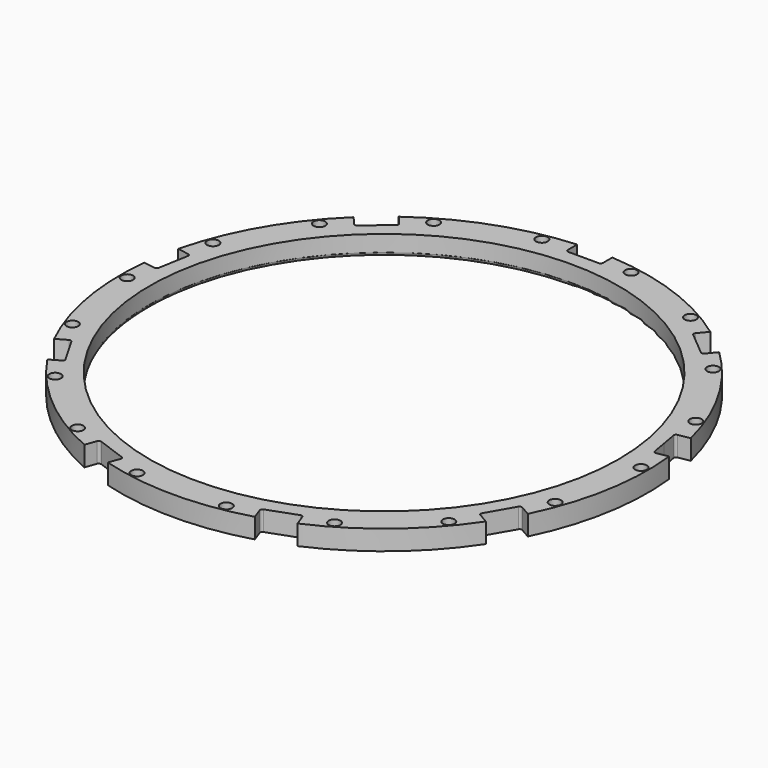
from build123d import *

# Parameters (mm, degrees)
F0_R           = 225
F0_R_2         = 200
F1_DEPTH       = 17
F3_D           = 5.5
F3_CBORE_D     = 10
F3_CBORE_DEPTH = 5.4
F4_R           = 3
F6_DEPTH       = 17.001


# Not quite as in the source:
# - a feature names something its author has since deleted; it is built from what else it names


with BuildPart() as f1:
    # F0 (on Top) → F1 (new body)
    with BuildSketch(Plane.XY):
        Circle(F0_R)
        Circle(F0_R_2, mode=Mode.SUBTRACT)
    extrude(amount=F1_DEPTH)

    # F3 (through all)
    with Locations(Plane.XY.offset(17)):
        with Locations((219, 0), (205.7926839521, 74.9024113883), (167.7637330431, 140.7704865214), (109.5, 189.6595634288), (38.0289509091, 215.6728979097), (-38.0289509091, 215.6728979097), (-109.5, 189.6595634288), (-167.7637330431, 140.7704865214), (-205.7926839521, 74.9024113883), (-219, 0), (-205.7926839521, -74.9024113883), (-167.7637330431, -140.7704865214), (-109.5, -189.6595634288), (-38.0289509091, -215.6728979097), (38.0289509091, -215.6728979097), (109.5, -189.6595634288), (167.7637330431, -140.7704865214), (205.7926839521, -74.9024113883)):
            CounterBoreHole(F3_D / 2, F3_CBORE_D / 2, F3_CBORE_DEPTH)

    # F4
    f4_edges = [f1.edges().sort_by_distance(p)[0] for p in [
        (-200, 0, 0),
    ]]
    fillet(f4_edges, radius=F4_R)

    # F5 (on face) → F6 (cut, through all)
    with BuildSketch(Plane.XY.offset(17)):
        with BuildLine():
            ThreePointArc((223.6935148816, 24.2118029049), (221.5817444277, 39.0708399751), (218.4840695516, 53.7560354952))
            Line((218.4840695516, 53.7560354952), (208.6359920215, 52.0195537186))
            ThreePointArc((208.6359920215, 52.0195537186), (207.3449842883, 51.1970910852), (207.0136728708, 49.7026418572))
            Line((207.0136728708, 49.7026418572), (209.2710991805, 36.900141068))
            Line((209.2710991805, 36.900141068), (211.5285254901, 24.0976402789))
            ThreePointArc((211.5285254901, 24.0976402789), (212.3509881235, 22.8066325456), (213.8454373515, 22.4753211282))
            Line((213.8454373515, 22.4753211282), (223.6935148816, 24.2118029049))
        make_face()
        with BuildLine():
            Line((149.3682510245, 154.6742923751), (155.7961271214, 162.3347368063))
            ThreePointArc((155.7961271214, 162.3347368063), (144.6272121795, 172.3599997018), (132.8147938278, 181.6183650969))
            Line((132.8147938278, 181.6183650969), (126.386917731, 173.9579206657))
            ThreePointArc((126.386917731, 173.9579206657), (125.926617221, 172.4980339608), (126.6334313978, 171.1402565601))
            Line((126.6334313978, 171.1402565601), (136.5920091584, 162.7840176342))
            Line((136.5920091584, 162.7840176342), (146.5505869189, 154.4277787082))
            ThreePointArc((146.5505869189, 154.4277787082), (148.0104736238, 153.9674781983), (149.3682510245, 154.6742923751))
        make_face()
        with BuildLine():
            Line((15, 214.4994432064), (15, 224.4994432064))
            ThreePointArc((15, 224.4994432064), (0, 225), (-15, 224.4994432064))
            Line((-15, 224.4994432064), (-15, 214.4994432064))
            ThreePointArc((-15, 214.4994432064), (-14.4142135624, 213.0852296441), (-13, 212.4994432064))
            Line((-13, 212.4994432064), (0, 212.4994432064))
            Line((0, 212.4994432064), (13, 212.4994432064))
            ThreePointArc((13, 212.4994432064), (14.4142135624, 213.0852296441), (15, 214.4994432064))
        make_face()
        with BuildLine():
            Line((-126.386917731, 173.9579206657), (-132.8147938278, 181.6183650969))
            ThreePointArc((-132.8147938278, 181.6183650969), (-144.6272121795, 172.3599997018), (-155.7961271214, 162.3347368063))
            Line((-155.7961271214, 162.3347368063), (-149.3682510245, 154.6742923751))
            ThreePointArc((-149.3682510245, 154.6742923751), (-148.0104736238, 153.9674781983), (-146.5505869189, 154.4277787082))
            Line((-146.5505869189, 154.4277787082), (-136.5920091584, 162.7840176342))
            Line((-136.5920091584, 162.7840176342), (-126.6334313978, 171.1402565601))
            ThreePointArc((-126.6334313978, 171.1402565601), (-125.926617221, 172.4980339608), (-126.386917731, 173.9579206657))
        make_face()
        with BuildLine():
            Line((-208.6359920215, 52.0195537186), (-218.4840695516, 53.7560354952))
            ThreePointArc((-218.4840695516, 53.7560354952), (-221.5817444277, 39.0708399751), (-223.6935148816, 24.2118029049))
            Line((-223.6935148816, 24.2118029049), (-213.8454373515, 22.4753211282))
            ThreePointArc((-213.8454373515, 22.4753211282), (-212.3509881235, 22.8066325456), (-211.5285254901, 24.0976402789))
            Line((-211.5285254901, 24.0976402789), (-209.2710991805, 36.900141068))
            Line((-209.2710991805, 36.900141068), (-207.0136728708, 49.7026418572))
            ThreePointArc((-207.0136728708, 49.7026418572), (-207.3449842883, 51.1970910852), (-208.6359920215, 52.0195537186))
        make_face()
        with BuildLine():
            ThreePointArc((-201.9222209522, -99.2593405465), (-194.8557158515, -112.5), (-186.9222209522, -125.24010266))
            Line((-186.9222209522, -125.24010266), (-178.2619669144, -120.24010266))
            ThreePointArc((-178.2619669144, -120.24010266), (-177.3301152618, -119.0256899426), (-177.5299161068, -117.5080518524))
            Line((-177.5299161068, -117.5080518524), (-184.0299161068, -106.2497216032))
            Line((-184.0299161068, -106.2497216032), (-190.5299161068, -94.991391354))
            ThreePointArc((-190.5299161068, -94.991391354), (-191.7443288242, -94.0595397014), (-193.2619669144, -94.2593405465))
            Line((-193.2619669144, -94.2593405465), (-201.9222209522, -99.2593405465))
        make_face()
        with BuildLine():
            ThreePointArc((-90.8787210538, -205.8301680017), (-76.9545322483, -211.4308396768), (-62.6879424302, -216.0907723015))
            Line((-62.6879424302, -216.0907723015), (-59.267740997, -206.6938460937))
            ThreePointArc((-59.267740997, -206.6938460937), (-59.3345106645, -205.1645692835), (-60.4630859519, -204.1304205654))
            Line((-60.4630859519, -204.1304205654), (-72.6790900221, -199.6841587022))
            Line((-72.6790900221, -199.6841587022), (-84.8950940923, -195.237896839))
            ThreePointArc((-84.8950940923, -195.237896839), (-86.4243709024, -195.3046665065), (-87.4585196205, -196.4332417939))
            Line((-87.4585196205, -196.4332417939), (-90.8787210538, -205.8301680017))
        make_face()
        with BuildLine():
            ThreePointArc((62.6879424302, -216.0907723015), (76.9545322483, -211.4308396768), (90.8787210538, -205.8301680017))
            Line((90.8787210538, -205.8301680017), (87.4585196205, -196.4332417939))
            ThreePointArc((87.4585196205, -196.4332417939), (86.4243709024, -195.3046665065), (84.8950940923, -195.237896839))
            Line((84.8950940923, -195.237896839), (72.6790900221, -199.6841587022))
            Line((72.6790900221, -199.6841587022), (60.4630859519, -204.1304205654))
            ThreePointArc((60.4630859519, -204.1304205654), (59.3345106645, -205.1645692835), (59.267740997, -206.6938460937))
            Line((59.267740997, -206.6938460937), (62.6879424302, -216.0907723015))
        make_face()
        with BuildLine():
            ThreePointArc((186.9222209522, -125.24010266), (194.8557158515, -112.5), (201.9222209522, -99.2593405465))
            Line((201.9222209522, -99.2593405465), (193.2619669144, -94.2593405465))
            ThreePointArc((193.2619669144, -94.2593405465), (191.7443288242, -94.0595397014), (190.5299161068, -94.991391354))
            Line((190.5299161068, -94.991391354), (184.0299161068, -106.2497216032))
            Line((184.0299161068, -106.2497216032), (177.5299161068, -117.5080518524))
            ThreePointArc((177.5299161068, -117.5080518524), (177.3301152618, -119.0256899426), (178.2619669144, -120.24010266))
            Line((178.2619669144, -120.24010266), (186.9222209522, -125.24010266))
        make_face()
    extrude(amount=-F6_DEPTH, mode=Mode.SUBTRACT)


solid = f1.part
